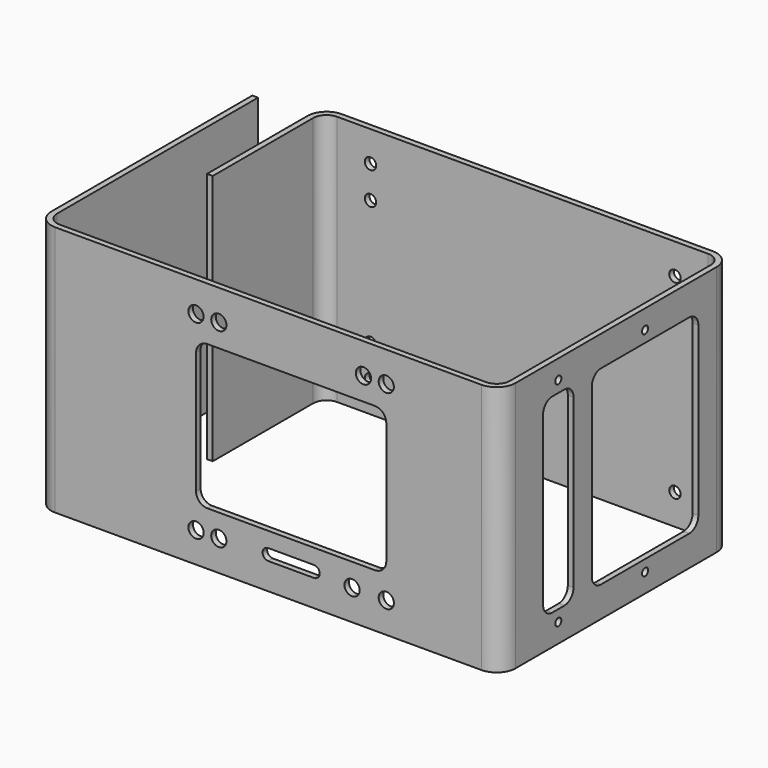
from build123d import *

# Parameters (mm, degrees)
F1_DEPTH = 66
F2_R     = 2
F3_DEPTH = 25
F4_R     = 1.5
F5_DEPTH = 25
F6_R     = 1
F7_DEPTH = 25


# Not quite as in the source:
# - a feature names something its author has since deleted; it is built from what else it names


with BuildPart() as f1:
    # F0 (on Top) → F1 (new body)
    with BuildSketch(Plane.XY):
        with BuildLine():
            Line((-66.75, -33), (-66.75, 33))
            Line((-66.75, 33), (-68.25, 33))
            Line((-68.25, 33), (-68.25, -33))
            ThreePointArc((-68.25, -33), (-66.7855339059, -36.5355339059), (-63.25, -38))
            Line((-63.25, -38), (48.75, -38))
            ThreePointArc((48.75, -38), (52.2855339059, -36.5355339059), (53.75, -33))
            Line((53.75, -33), (53.75, 33))
            ThreePointArc((53.75, 33), (52.2855339059, 36.5355339059), (48.75, 38))
            Line((48.75, 38), (-48.75, 38))
            ThreePointArc((-48.75, 38), (-52.2855339059, 36.5355339059), (-53.75, 33))
            Line((-53.75, 33), (-53.75, 0))
            Line((-53.75, 0), (-52.25, 0))
            Line((-52.25, 0), (-52.25, 33))
            ThreePointArc((-52.25, 33), (-51.2248737342, 35.4748737342), (-48.75, 36.5))
            Line((-48.75, 36.5), (48.75, 36.5))
            ThreePointArc((48.75, 36.5), (51.2248737342, 35.4748737342), (52.25, 33))
            Line((52.25, 33), (52.25, -33))
            ThreePointArc((52.25, -33), (51.2248737342, -35.4748737342), (48.75, -36.5))
            Line((48.75, -36.5), (-63.25, -36.5))
            ThreePointArc((-63.25, -36.5), (-65.7248737342, -35.4748737342), (-66.75, -33))
        make_face()
    extrude(amount=F1_DEPTH)

    # F2 (on face) → F3 (cut)
    with BuildSketch(Plane.XZ.offset(38)):
        with BuildLine():
            Line((20.75, 52), (-23.25, 52))
            ThreePointArc((-23.25, 52), (-25.3713203436, 51.1213203436), (-26.25, 49))
            Line((-26.25, 49), (-26.25, 17))
            ThreePointArc((-26.25, 17), (-25.3713203436, 14.8786796564), (-23.25, 14))
            Line((-23.25, 14), (20.75, 14))
            ThreePointArc((20.75, 14), (22.8713203436, 14.8786796564), (23.75, 17))
            Line((23.75, 17), (23.75, 49))
            ThreePointArc((23.75, 49), (22.8713203436, 51.1213203436), (20.75, 52))
        make_face()
        with Locations((-26.25, 58)):
            Circle(F2_R)
        with Locations((23.75, 58)):
            Circle(F2_R)
        with Locations((23.75, 8)):
            Circle(F2_R)
        with Locations((-26.25, 8)):
            Circle(F2_R)
        with BuildLine():
            ThreePointArc((-8.75, 8.5), (-8.3106601718, 7.4393398282), (-7.25, 7))
            Line((-7.25, 7), (4.75, 7))
            ThreePointArc((4.75, 7), (5.8106601718, 7.4393398282), (6.25, 8.5))
            ThreePointArc((6.25, 8.5), (5.8106601718, 9.5606601718), (4.75, 10))
            Line((4.75, 10), (-7.25, 10))
            ThreePointArc((-7.25, 10), (-8.3106601718, 9.5606601718), (-8.75, 8.5))
        make_face()
        with Locations((-20.25, 8)):
            Circle(F2_R)
        with Locations((-20.25, 58)):
            Circle(F2_R)
        with Locations((17.75, 58)):
            Circle(F2_R)
        with Locations((14.75, 8)):
            Circle(F2_R)
    extrude(amount=-F3_DEPTH, mode=Mode.SUBTRACT)

    # F4 (on face) → F5 (cut)
    with BuildSketch(Plane(origin=(0, 38, 0), x_dir=(-1, 0, 0), z_dir=(0, 1, 0))):
        with Locations((-40, 58)):
            Circle(F4_R)
        with Locations((-40, 8)):
            Circle(F4_R)
        with Locations((40, 8)):
            Circle(F4_R)
        with Locations((40, 58)):
            Circle(F4_R)
        with Locations((40, 16.5)):
            Circle(F4_R)
        with Locations((40, 49.5)):
            Circle(F4_R)
    extrude(amount=-F5_DEPTH, mode=Mode.SUBTRACT)

    # F6 (on face) → F7 (cut)
    with BuildSketch(Plane.YZ.offset(53.75)):
        with BuildLine():
            Line((-17, 58), (-21, 58))
            ThreePointArc((-21, 58), (-23.1213203436, 57.1213203436), (-24, 55))
            Line((-24, 55), (-24, 11))
            ThreePointArc((-24, 11), (-23.1213203436, 8.8786796564), (-21, 8))
            Line((-21, 8), (-17, 8))
            ThreePointArc((-17, 8), (-14.8786796564, 8.8786796564), (-14, 11))
            Line((-14, 11), (-14, 55))
            ThreePointArc((-14, 55), (-14.8786796564, 57.1213203436), (-17, 58))
        make_face()
        with BuildLine():
            Line((24, 58), (-5, 58))
            ThreePointArc((-5, 58), (-7.1213203436, 57.1213203436), (-8, 55))
            Line((-8, 55), (-8, 11))
            ThreePointArc((-8, 11), (-7.1213203436, 8.8786796564), (-5, 8))
            Line((-5, 8), (24, 8))
            ThreePointArc((24, 8), (26.1213203436, 8.8786796564), (27, 11))
            Line((27, 11), (27, 55))
            ThreePointArc((27, 55), (26.1213203436, 57.1213203436), (24, 58))
        make_face()
        with Locations((-19, 61)):
            Circle(F6_R)
        with Locations((9.5, 61)):
            Circle(F6_R)
        with Locations((9.5, 5)):
            Circle(F6_R)
        with Locations((-19, 5)):
            Circle(F6_R)
    extrude(amount=-F7_DEPTH, mode=Mode.SUBTRACT)


solid = f1.part
